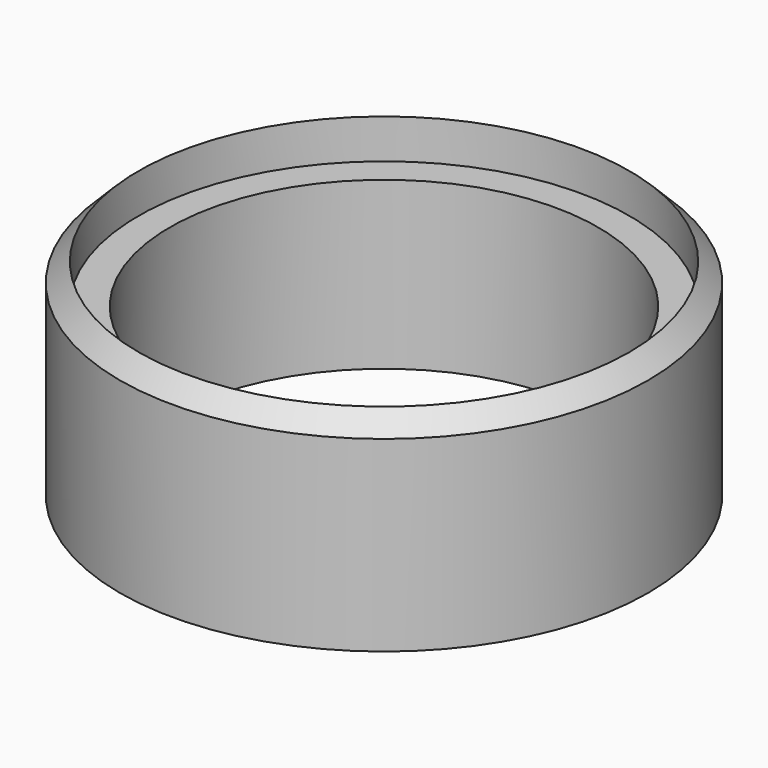
from build123d import *

# Parameters (mm, degrees)
F0_R     = 6.35
F0_R_2   = 5.15
F1_DEPTH = 5
F2_R     = 5.9
F2_R_2   = 5.15
F3_DEPTH = 1


# Not quite as in the source:
# - a fillet or chamfer that OpenCascade refuses, or shapes differently, is made with other operations: its cross-section is extruded or revolved along the edge and cut away or added


with BuildPart() as f1:
    # F0 (on Top) → F1 (new body)
    with BuildSketch(Plane.XY):
        Circle(F0_R)
        Circle(F0_R_2, mode=Mode.SUBTRACT)
    extrude(amount=F1_DEPTH)

    # F2 (on face) → F3 (cut)
    with BuildSketch(Plane.XY.offset(5)):
        Circle(F2_R)
        Circle(F2_R_2, mode=Mode.SUBTRACT)
    extrude(amount=-F3_DEPTH, mode=Mode.SUBTRACT)

    # F4: chamfer of 0.5 on 1 edges, made by hand

    # F4_s1 → F4_t2 (revolve, cut)
    with BuildSketch(Plane.XZ):
        Polygon((6.35, 4.5), (5.85, 5), (6.35, 5), align=None)
    revolve(axis=Axis((0, 0, 5), (0, 0, 1)), mode=Mode.SUBTRACT)


solid = f1.part
